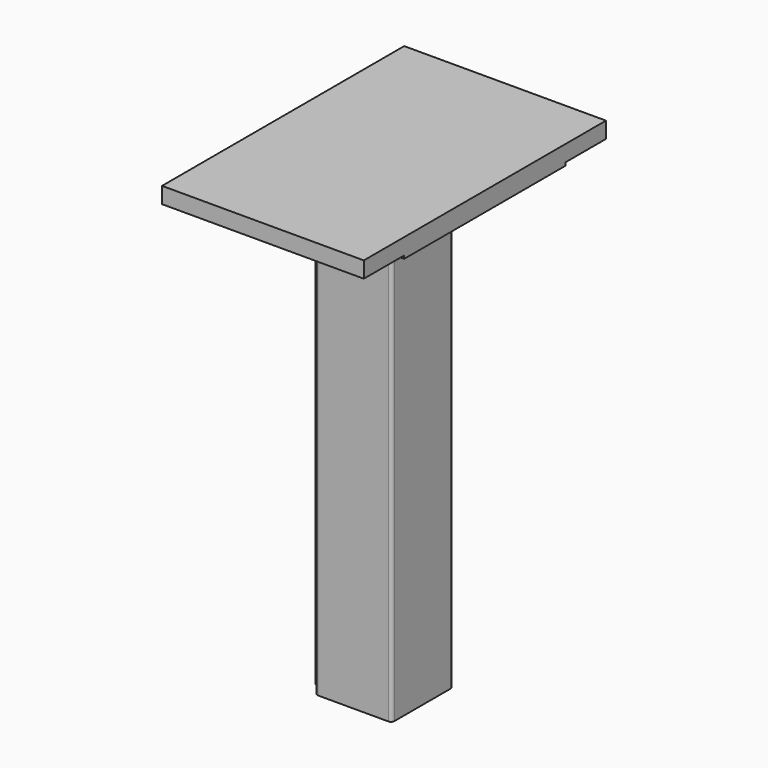
from build123d import *

# Parameters (mm, degrees)
F0_W     = 70.104
F0_H     = 70.104
F1_DEPTH = 450
F2_W     = 50
F2_H     = 370
F3_DEPTH = 10
F4_W     = 200
F4_H     = 300
F5_DEPTH = 19
F6_W     = 50
F6_H     = 3
F7_DEPTH = 254


with BuildPart() as f1:
    # F0 (on Top) → F1 (new body)
    with BuildSketch(Plane.XY):
        with BuildLine():
            Line((34.925, 38.1), (-34.925, 38.1))
            ThreePointArc((-34.925, 38.1), (-37.1700640303, 37.1700640303), (-38.1, 34.925))
            Line((-38.1, 34.925), (-38.1, -34.925))
            ThreePointArc((-38.1, -34.925), (-37.1700640303, -37.1700640303), (-34.925, -38.1))
            Line((-34.925, -38.1), (34.925, -38.1))
            ThreePointArc((34.925, -38.1), (37.1700640303, -37.1700640303), (38.1, -34.925))
            Line((38.1, -34.925), (38.1, 34.925))
            ThreePointArc((38.1, 34.925), (37.1700640303, 37.1700640303), (34.925, 38.1))
        make_face()
        Rectangle(F0_W, F0_H, mode=Mode.SUBTRACT)
    extrude(amount=-F1_DEPTH)

    # F2 (on face) → F3 (join)
    with BuildSketch(Plane(origin=(-38.1, 0, 0), x_dir=(0, -1, 0), z_dir=(-1, 0, 0))):
        with Locations((0, -265)):
            Rectangle(F2_W, F2_H)
    extrude(amount=F3_DEPTH)

    # F4 (on Top) → F5 (join)
    with BuildSketch(Plane.XY):
        Rectangle(F4_W, F4_H)
    extrude(amount=F5_DEPTH)

    # F6 (on face) → F7 (cut)
    with BuildSketch(Plane(origin=(-100, 0, 0), x_dir=(0, -1, 0), z_dir=(-1, 0, 0))):
        with Locations((125, 1.5)):
            Rectangle(F6_W, F6_H)
        with Locations((-125, 1.5)):
            Rectangle(F6_W, F6_H)
    extrude(amount=-F7_DEPTH, mode=Mode.SUBTRACT)


solid = f1.part
